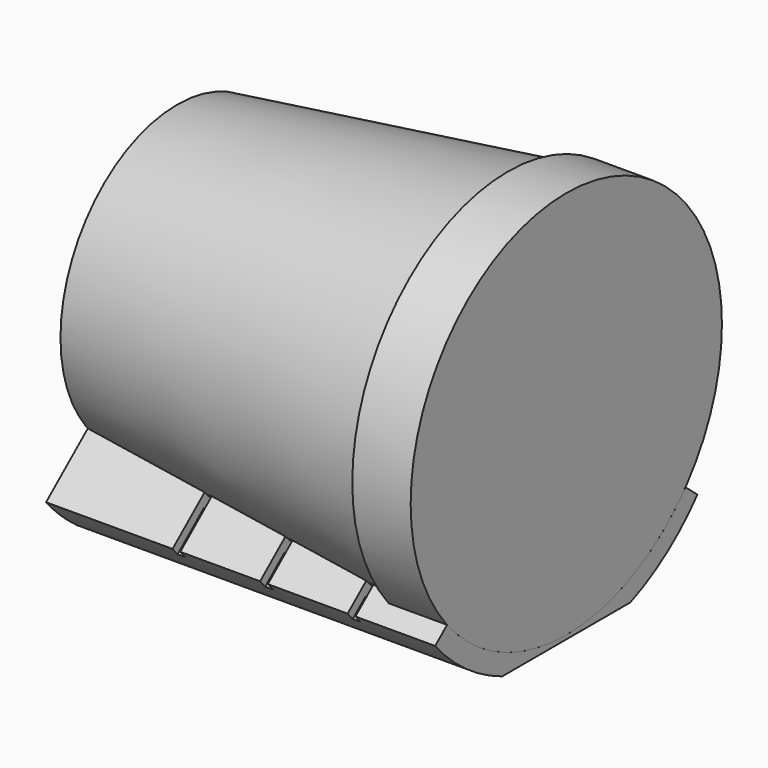
from build123d import *

# Parameters (mm, degrees)
F0_R          = 37.5
F2_R          = 50
F4_R          = 50
F6_DEPTH      = 15
F7_DEPTH      = 10
F9_ANGLE_BACK = 50
F9_ANGLE      = 100
F10_W         = 2
F10_H         = 2.5
F11_ANGLE     = 100
F13_DEPTH     = 100
F14_W         = 2
F14_H         = 10.9375
F14_H_2       = 8.125
F14_H_3       = 5.3125
F15_DEPTH     = 2.5
F16_W         = 2
F16_H         = 5.3125
F16_H_2       = 8.125
F16_H_3       = 10.9375
F17_DEPTH     = 2.5


# Not quite as in the source:
# - a feature names something its author has since deleted; it is built from what else it names


with BuildPart() as f5:
    # F0 (on Right) → F5 section 0
    with BuildSketch(Plane.YZ):
        Circle(F0_R)
    # F2 (on offset) → F5 section 1
    with BuildSketch(Plane.YZ.offset(100)):
        Circle(F2_R)
    loft()

    # F4 (on offset) → F6 (join, through all)
    with BuildSketch(Plane.YZ.offset(85)):
        Circle(F4_R)
    extrude(amount=F6_DEPTH)

    # F7 (cut): a face of the model
    f7_faces = [f5.faces().sort_by_distance(p)[0] for p in [
        (0, 0, 0),
    ]]
    extrude(f7_faces, amount=-F7_DEPTH, mode=Mode.SUBTRACT)


with BuildPart() as f9:
    # F8 (on Front) → F9 (revolve)
    with BuildSketch(Plane.XZ, mode=Mode.PRIVATE) as f9_sk:
        Polygon((85, -50), (85, -48.125), (0, -37.5), (0, -55), (100, -55), (100, -50), align=None)
    revolve(f9_sk.sketch.rotate(Axis((53.7593327463, 0, 0), (1, 0, 0)), -F9_ANGLE_BACK), axis=Axis((53.7593327463, 0, 0), (1, 0, 0)), revolution_arc=F9_ANGLE)


with BuildPart() as f11_tool:
    # F10 (on face) → F11 (revolve)
    with BuildSketch(Plane(origin=(0, 0, 0), x_dir=(1, 0, 0), z_dir=(0, -0.6427876097, 0.7660444431))):
        with Locations((33.5, -42.8125)):
            Rectangle(F10_W, F10_H)
        with Locations((56, -45.625)):
            Rectangle(F10_W, F10_H)
        with Locations((78.5, -48.4375)):
            Rectangle(F10_W, F10_H)
    revolve(axis=Axis((53.7593327463, 0, 0), (1, 0, 0)), revolution_arc=F11_ANGLE)


with BuildPart() as f5_1:
    add(f5.part)

    # F11: cut by f11_tool
    add(f11_tool.part, mode=Mode.SUBTRACT)


with BuildPart() as f9_1:
    add(f9.part)

    # F11: cut by f11_tool
    add(f11_tool.part, mode=Mode.SUBTRACT)

    # F12 (on face) → F13 (cut, through all)
    with BuildSketch(Plane.YZ.offset(100)):
        with BuildLine():
            Line((-20.591260282, -51), (-50.5514740944, -51))
            Line((-50.5514740944, -51), (-50.5514740944, -60.0057376325))
            Line((-50.5514740944, -60.0057376325), (49.9166063964, -60.0057376325))
            Line((49.9166063964, -60.0057376325), (49.9166063964, -51))
            Line((49.9166063964, -51), (20.591260282, -51))
            ThreePointArc((20.591260282, -51), (0, -55), (-20.591260282, -51))
        make_face()
        with BuildLine():
            Line((20.591260282, -51), (-20.591260282, -51))
            ThreePointArc((-20.591260282, -51), (0, -55), (20.591260282, -51))
        make_face()
    extrude(amount=-F13_DEPTH, mode=Mode.SUBTRACT)

    # F14 (on face) → F15 (cut)
    with BuildSketch(Plane(origin=(0, 0, 0), x_dir=(1, 0, 0), z_dir=(0, -0.6427876097, 0.7660444431))):
        with Locations((33.5, -49.53125)):
            Rectangle(F14_W, F14_H)
        Polygon((34.5, -41.5625), (32.5, -41.5625), (32.5, -44.0625), (34.5, -44.0625), (34.5, -41.8125), align=None)
        Polygon((57, -44.375), (55, -44.375), (55, -46.875), (57, -46.875), (57, -44.625), align=None)
        with Locations((56, -50.9375)):
            Rectangle(F14_W, F14_H_2)
        Polygon((79.5, -47.1875), (77.5, -47.1875), (77.5, -49.6875), (79.5, -49.6875), (79.5, -47.4375), align=None)
        with Locations((78.5, -52.34375)):
            Rectangle(F14_W, F14_H_3)
    extrude(amount=-F15_DEPTH, mode=Mode.SUBTRACT)

    # F16 (on face) → F17 (cut)
    with BuildSketch(Plane(origin=(0, 0, 0), x_dir=(1, 0, 0), z_dir=(0, 0.6427876097, 0.7660444431))):
        with Locations((78.5, 52.34375)):
            Rectangle(F16_W, F16_H)
        Polygon((77.5, 49.6875), (77.5, 47.1875), (79.5, 47.1875), (79.5, 47.4375), (79.5, 49.6875), align=None)
        Polygon((55, 46.875), (55, 44.375), (57, 44.375), (57, 44.625), (57, 46.875), align=None)
        with Locations((56, 50.9375)):
            Rectangle(F16_W, F16_H_2)
        with Locations((33.5, 49.53125)):
            Rectangle(F16_W, F16_H_3)
        Polygon((32.5, 44.0625), (32.5, 41.5625), (34.5, 41.5625), (34.5, 41.8125), (34.5, 44.0625), align=None)
    extrude(amount=-F17_DEPTH, mode=Mode.SUBTRACT)


solid = Compound([f5_1.part, f9_1.part])
